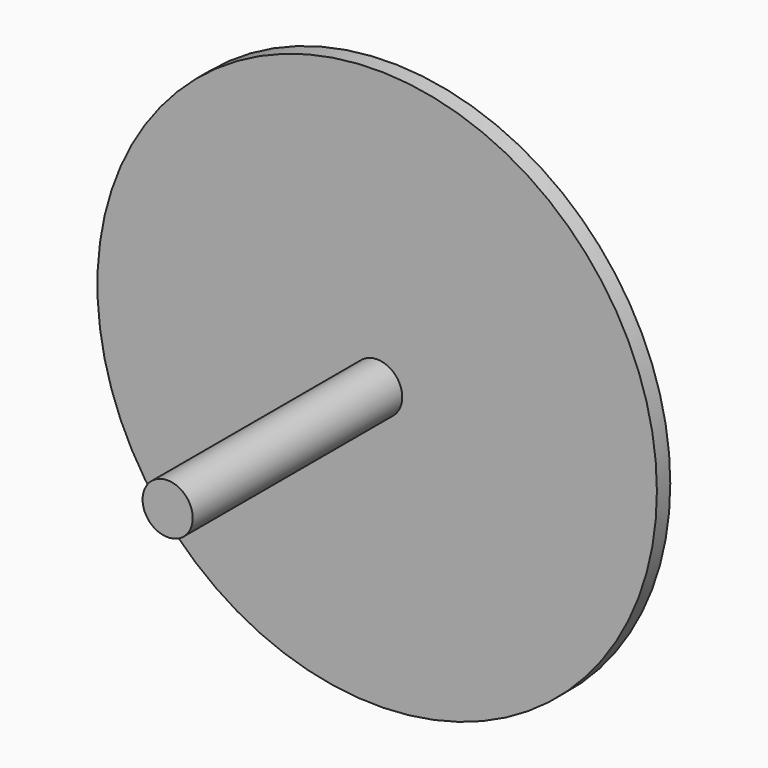
from build123d import *

# Parameters (mm, degrees)
F0_R     = 50.2
F0_R_2   = 4.5
F1_DEPTH = 3
F4_R     = 4.5
F5_DEPTH = 50


# Not quite as in the source:
# - the program builds the solid bodies; features that only make, move or delete a surface that nothing else refers to are left out


with BuildPart() as f1:
    # F0 (on Front) → F1 (new body)
    with BuildSketch(Plane.XZ):
        Circle(F0_R)
        Circle(F0_R_2, mode=Mode.SUBTRACT)
    extrude(amount=F1_DEPTH)

    # F4 (on Front) → F5 (join)
    with BuildSketch(Plane.XZ):
        Circle(F4_R)
    extrude(amount=F5_DEPTH)


solid = f1.part
